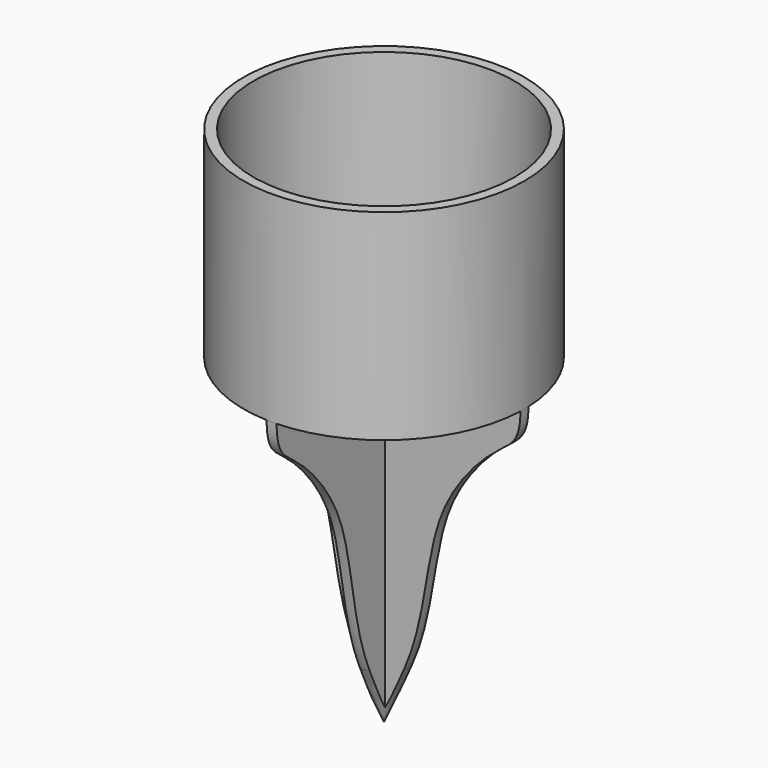
from build123d import *

# Parameters (mm, degrees)
F2_W         = 65.4981237411
F2_H         = 65.4981237411
F2_H_2       = 68.2687636971
F3_DEPTH     = 101.6
F4_R         = 44.45
F5_DEPTH     = 63.5
F6_T         = 3.175
F6_T3_DEPTH  = 49.1841427403
F6_T5_DEPTH  = 102.8165560233
F6_T7_DEPTH  = 49.1841427403
F6_T9_DEPTH  = 49.1841427403
F6_T11_DEPTH = 49.1841427403


# Not quite as in the source:
# - a shell that OpenCascade refuses in one call is made with other operations: the cavity is built on its own and cut out


with BuildPart() as f1:
    # F0 (on Front) → F1 (revolve)
    with BuildSketch(Plane.XZ):
        with BuildLine():
            Line((0, 101.6), (0, 0))
            Line((0, 0), (7.7969783843, 17.828155983))
            add(Edge.make_bspline(
                [(7.7969783843, 17.828155983), (14.8930814395, 34.0537277243), (13.801273804, 64.5218843491), (36.8201349812, 89.6629422756), (44.45, 92.7033537653), (44.45, 101.6)],
                knots=[0, 0, 0, 0, 0.4271461897, 0.75929401, 1, 1, 1, 1], degree=3))
            Line((44.45, 101.6), (0, 101.6))
        make_face()
    revolve(axis=Axis((0, 0, 50.8), (0, 0, -1)))

    # F2 (on Top) → F3 (cut, through all)
    with BuildSketch(Plane.XY):
        with Locations((-34.3365618706, -34.3365618706)):
            Rectangle(F2_W, F2_H)
        with Locations((34.3365618706, 35.7218818486)):
            Rectangle(F2_W, F2_H_2)
        with Locations((-34.3365618706, 35.7218818486)):
            Rectangle(F2_W, F2_H_2)
        with Locations((34.3365618706, -34.3365618706)):
            Rectangle(F2_W, F2_H)
    extrude(amount=F3_DEPTH, mode=Mode.SUBTRACT)

    # F4 (on face) → F5 (join)
    with BuildSketch(Plane.XY.offset(101.6)):
        Circle(F4_R)
    extrude(amount=F5_DEPTH)

    # F6: shell of thickness 3.175, made by hand


with BuildPart() as f6_core1:
    # F6_t2: copy of F1
    add(f1.part)

    # the walls: a layer under each face that stays
    f6_faces = [f6_core1.faces().sort_by_distance(p)[0] for p in [
        (22.6899295983, 0, 71.3288999003),
        (-44.45, 0, 133.35),
        (8.7265237901, 1.5875, 85.5222406628),
        (-3.8984891922, 0, 8.9140779915),
        (23.0045713702, -1.5875, 85.5222406628),
        (23.0045713702, 23.0045713702, 101.6),
        (0, 22.6899295983, 71.3288999003),
        (-23.0045713702, 23.0045713702, 101.6),
        (-22.6899295983, 0, 71.3288999003),
        (-23.0045713702, -23.0045713702, 101.6),
        (0, -22.6899295983, 71.3288999003),
        (23.0045713702, -23.0045713702, 101.6),
        (1.5875, 23.0045713702, 85.5222406628),
        (1.5875, -8.7265237901, 85.5222406628),
        (-1.5875, -23.0045713702, 85.5222406628),
        (-8.7265237901, -1.5875, 85.5222406628),
        (-23.0045713702, 1.5875, 85.5222406628),
        (-1.5875, 8.7265237901, 85.5222406628),
    ]]
    thicken(f6_faces, amount=-F6_T, mode=Mode.SUBTRACT)

    # F6_s4 → F6_t3 (cut)
    with BuildSketch(Plane.YZ.offset(-1.5875)):
        Polygon((1.61925, 101.56825), (-1.5875, 101.6), (-1.5875, 104.775), (1.5875, 104.775), align=None)
        Polygon((-1.61925, 101.56825), (1.5875, 101.6), (1.5875, 104.775), (-1.5875, 104.775), align=None)
    extrude(amount=F6_T3_DEPTH, mode=Mode.SUBTRACT)

    # F6_s6 → F6_t5 (cut)
    with BuildSketch(Plane.XY.offset(1.9584439767)):
        Polygon((1.61925, 1.61925), (1.5875, -1.5875), (-1.5875, -1.5875), (-1.5875, 1.5875), align=None)
        Polygon((1.61925, -1.61925), (1.5875, 1.5875), (-1.5875, 1.5875), (-1.5875, -1.5875), align=None)
        Polygon((-1.61925, -1.61925), (1.5875, -1.5875), (1.5875, 1.5875), (-1.5875, 1.5875), align=None)
        Polygon((-1.61925, 1.61925), (-1.5875, -1.5875), (1.5875, -1.5875), (1.5875, 1.5875), align=None)
    extrude(amount=F6_T5_DEPTH, mode=Mode.SUBTRACT)

    # F6_s8 → F6_t7 (cut)
    with BuildSketch(Plane.XZ.offset(-47.5966427403)):
        Polygon((1.61925, 101.56825), (1.5875, 104.775), (-1.5875, 104.775), (-1.5875, 101.6), align=None)
        Polygon((-1.61925, 101.56825), (-1.5875, 104.775), (1.5875, 104.775), (1.5875, 101.6), align=None)
    extrude(amount=F6_T7_DEPTH, mode=Mode.SUBTRACT)

    # F6_s10 → F6_t9 (cut)
    with BuildSketch(Plane.YZ.offset(-47.5966427403)):
        Polygon((1.61925, 101.56825), (1.5875, 104.775), (-1.5875, 104.775), (-1.5875, 101.6), align=None)
        Polygon((-1.61925, 101.56825), (-1.5875, 104.775), (1.5875, 104.775), (1.5875, 101.6), align=None)
    extrude(amount=F6_T9_DEPTH, mode=Mode.SUBTRACT)

    # F6_s12 → F6_t11 (cut)
    with BuildSketch(Plane.XZ.offset(-1.5875)):
        Polygon((-1.61925, 101.56825), (-1.5875, 104.775), (1.5875, 104.775), (1.5875, 101.6), align=None)
        Polygon((1.61925, 101.56825), (1.5875, 104.775), (-1.5875, 104.775), (-1.5875, 101.6), align=None)
    extrude(amount=F6_T11_DEPTH, mode=Mode.SUBTRACT)


with BuildPart() as f1_1:
    add(f1.part)

    # what is left inside the walls is the cavity
    f6_cavity = [f6_core1.part.solids().sort_by_distance(p)[0] for p in [
        (-41.24325, 0, 144.991667),
    ]]
    add(f6_cavity, mode=Mode.SUBTRACT)


solid = f1_1.part
